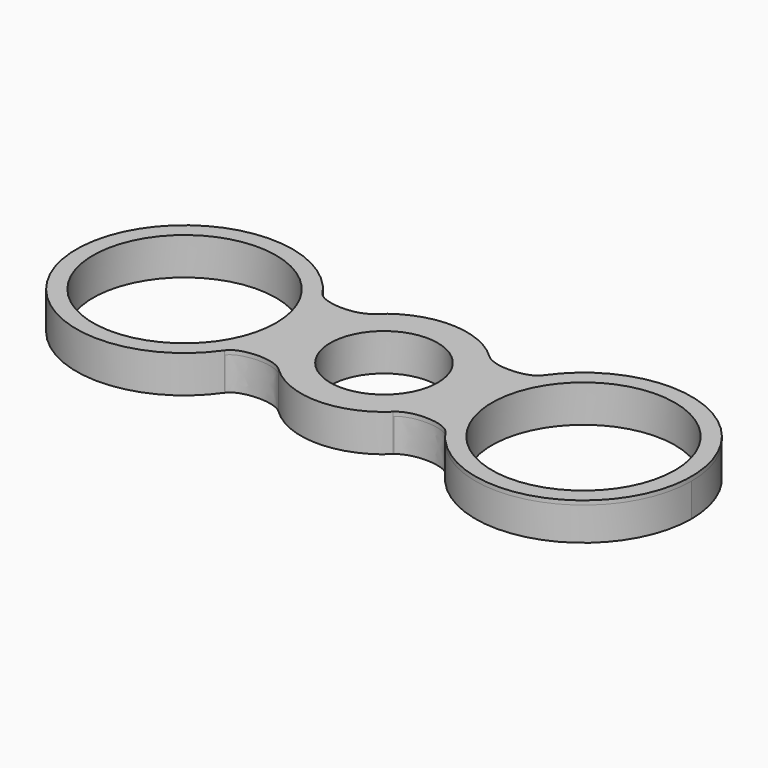
from build123d import *

# Parameters (mm, degrees)
F0_R        = 11.025
F0_R_2      = 8
F0_R_3      = 6.475
F1_DEPTH    = 4
F2_DEPTH    = 4.5
F1_FACE_R   = 11.025
F1_FACE_R_2 = 8
F3_DEPTH    = 0.5


# Not quite as in the source:
# - a feature names something its author has since deleted; it is built from what else it names


with BuildPart() as f1:
    # F0 (on Top) → F1 (new body)
    with BuildSketch(Plane.XY):
        with BuildLine():
            add(Edge.make_bspline(
                [(-13.2970699227, 7.3866190681), (-13.2858031983, 7.3692786835), (-13.2740607617, 7.352142708), (-13.2618542065, 7.3352108101)],
                knots=[0, 0, 0, 0, 0.0117546856, 0.0117546856, 0.0117546856, 0.0117546856], degree=3))
            ThreePointArc((-13.2970699227, 7.3866190681), (-37.05, 0), (-13.2970699227, -7.3866190681))
            add(Edge.make_bspline(
                [(-13.2970699227, -7.3866190681), (-13.2858031983, -7.3692786835), (-13.2740607617, -7.352142708), (-13.2618542065, -7.3352108101)],
                knots=[0, 0, 0, 0, 0.0117546856, 0.0117546856, 0.0117546856, 0.0117546856], degree=3))
            ThreePointArc((-13.2618542065, -7.3352108101), (-11.5783016635, -3.8380106201), (-11, 0))
            ThreePointArc((-11, 0), (-11.5783016635, 3.8380106201), (-13.2618542065, 7.3352108101))
        make_face()
        with Locations((-24.025, 0)):
            Circle(F0_R, mode=Mode.SUBTRACT)
        with BuildLine():
            add(Edge.make_bspline(
                [(13.2970699227, 7.3866190681), (13.2858031983, 7.3692786835), (13.2740607617, 7.352142708), (13.2618542065, 7.3352108101)],
                knots=[0, 0, 0, 0, 0.0117546856, 0.0117546856, 0.0117546856, 0.0117546856], degree=3))
            ThreePointArc((13.2618542065, 7.3352108101), (11, 0), (13.2618542065, -7.3352108101))
            add(Edge.make_bspline(
                [(13.2970699227, -7.3866190681), (13.2858031983, -7.3692786835), (13.2740607617, -7.352142708), (13.2618542065, -7.3352108101)],
                knots=[0, 0, 0, 0, 0.0117546856, 0.0117546856, 0.0117546856, 0.0117546856], degree=3))
            ThreePointArc((13.2970699227, -7.3866190681), (27.8927729861, -12.4374819448), (37.05, 0))
            ThreePointArc((37.05, 0), (27.8927729861, 12.4374819448), (13.2970699227, 7.3866190681))
        make_face()
        with Locations((24.025, 0)):
            Circle(F0_R, mode=Mode.SUBTRACT)
        with BuildLine():
            add(Edge.make_bspline(
                [(-6.9491121946, 7.1909554099), (-6.9214787847, 7.2161071506), (-6.8945995038, 7.2417846871), (-6.8685019311, 7.2679901776)],
                knots=[0.9815772058, 0.9815772058, 0.9815772058, 0.9815772058, 1, 1, 1, 1], degree=3))
            ThreePointArc((-6.9491121946, 7.1909554099), (-10, 0), (-6.9491121946, -7.1909554099))
            add(Edge.make_bspline(
                [(-6.9491121946, -7.1909554099), (-6.9214787847, -7.2161071506), (-6.8945995038, -7.2417846871), (-6.8685019311, -7.2679901776)],
                knots=[0.9815772058, 0.9815772058, 0.9815772058, 0.9815772058, 1, 1, 1, 1], degree=3))
            ThreePointArc((-6.8685019311, -7.2679901776), (0, -10), (6.8685019311, -7.2679901776))
            add(Edge.make_bspline(
                [(6.9491121946, -7.1909554099), (6.9214787847, -7.2161071506), (6.8945995038, -7.2417846871), (6.8685019311, -7.2679901776)],
                knots=[0.9815772058, 0.9815772058, 0.9815772058, 0.9815772058, 1, 1, 1, 1], degree=3))
            ThreePointArc((6.9491121946, -7.1909554099), (9.2057352217, -3.9056931558), (10, 0))
            ThreePointArc((10, 0), (9.2057352217, 3.9056931558), (6.9491121946, 7.1909554099))
            add(Edge.make_bspline(
                [(6.9491121946, 7.1909554099), (6.9214787847, 7.2161071506), (6.8945995038, 7.2417846871), (6.8685019311, 7.2679901776)],
                knots=[0.9815772058, 0.9815772058, 0.9815772058, 0.9815772058, 1, 1, 1, 1], degree=3))
            ThreePointArc((6.8685019311, 7.2679901776), (0, 10), (-6.8685019311, 7.2679901776))
        make_face()
        Circle(F0_R_2, mode=Mode.SUBTRACT)
        Circle(F0_R_2)
        Circle(F0_R_3, mode=Mode.SUBTRACT)
        with BuildLine():
            add(Edge.make_bspline(
                [(-13.2618542065, 7.3352108101), (-12.765654406, 6.6469245328), (-10.2019626219, 5.934402015), (-7.687078337, 6.5192636743), (-6.9491121946, 7.1909554099)],
                knots=[0.0117546856, 0.0117546856, 0.0117546856, 0.0117546856, 0.4895858662, 0.9815772058, 0.9815772058, 0.9815772058, 0.9815772058], degree=3))
            ThreePointArc((-13.2618542065, 7.3352108101), (-11.5783016635, 3.8380106201), (-11, 0))
            ThreePointArc((-11, 0), (-11.5783016635, -3.8380106201), (-13.2618542065, -7.3352108101))
            add(Edge.make_bspline(
                [(-13.2618542065, -7.3352108101), (-12.765654406, -6.6469245328), (-10.2019626219, -5.934402015), (-7.687078337, -6.5192636743), (-6.9491121946, -7.1909554099)],
                knots=[0.0117546856, 0.0117546856, 0.0117546856, 0.0117546856, 0.4895858662, 0.9815772058, 0.9815772058, 0.9815772058, 0.9815772058], degree=3))
            ThreePointArc((-6.9491121946, -7.1909554099), (-10, 0), (-6.9491121946, 7.1909554099))
        make_face()
        with BuildLine():
            add(Edge.make_bspline(
                [(13.2618542065, 7.3352108101), (12.765654406, 6.6469245328), (10.2019626219, 5.934402015), (7.687078337, 6.5192636743), (6.9491121946, 7.1909554099)],
                knots=[0.0117546856, 0.0117546856, 0.0117546856, 0.0117546856, 0.4895858662, 0.9815772058, 0.9815772058, 0.9815772058, 0.9815772058], degree=3))
            ThreePointArc((6.9491121946, 7.1909554099), (9.2057352217, 3.9056931558), (10, 0))
            ThreePointArc((10, 0), (9.2057352217, -3.9056931558), (6.9491121946, -7.1909554099))
            add(Edge.make_bspline(
                [(13.2618542065, -7.3352108101), (12.765654406, -6.6469245328), (10.2019626219, -5.934402015), (7.687078337, -6.5192636743), (6.9491121946, -7.1909554099)],
                knots=[0.0117546856, 0.0117546856, 0.0117546856, 0.0117546856, 0.4895858662, 0.9815772058, 0.9815772058, 0.9815772058, 0.9815772058], degree=3))
            ThreePointArc((13.2618542065, -7.3352108101), (11, 0), (13.2618542065, 7.3352108101))
        make_face()
    extrude(amount=F1_DEPTH)

    # F0 (on Top) → F2 (join)
    with BuildSketch(Plane.XY):
        Circle(F0_R_2)
        Circle(F0_R_3, mode=Mode.SUBTRACT)
    extrude(amount=F2_DEPTH)

    # F1_face (on face) + F0 (on Top) → F3 (join, through all)
    with BuildSketch(Plane.XY.offset(4)):
        with BuildLine():
            ThreePointArc((-6.8685019311, -7.2679901776), (0, -10), (6.8685019311, -7.2679901776))
            add(Edge.make_bspline(
                [(6.8685019311, -7.2679901776), (7.591550229, -6.5419519543), (10.1837329047, -5.9134794065), (12.8278077735, -6.6643873129), (13.2970699227, -7.3866190681)],
                knots=[0.9815772058, 0.9815772058, 0.9815772058, 0.9815772058, 1.4919913396, 1.9815772058, 1.9815772058, 1.9815772058, 1.9815772058], degree=3))
            ThreePointArc((13.2970699227, -7.3866190681), (37.05, 0), (13.2970699227, 7.3866190681))
            add(Edge.make_bspline(
                [(13.2970699227, 7.3866190681), (12.8278077735, 6.6643873129), (10.1837329047, 5.9134794065), (7.591550229, 6.5419519543), (6.8685019311, 7.2679901776)],
                knots=[0, 0, 0, 0, 0.4895858662, 1, 1, 1, 1], degree=3))
            ThreePointArc((6.8685019311, 7.2679901776), (0, 10), (-6.8685019311, 7.2679901776))
            add(Edge.make_bspline(
                [(-6.8685019311, 7.2679901776), (-7.591550229, 6.5419519543), (-10.1837329047, 5.9134794066), (-12.8278077735, 6.6643873129), (-13.2970699227, 7.3866190681)],
                knots=[0.9815772058, 0.9815772058, 0.9815772058, 0.9815772058, 1.4919913396, 1.9815772058, 1.9815772058, 1.9815772058, 1.9815772058], degree=3))
            ThreePointArc((-13.2970699227, 7.3866190681), (-37.05, 0), (-13.2970699227, -7.3866190681))
            add(Edge.make_bspline(
                [(-13.2970699227, -7.3866190681), (-12.8278077735, -6.6643873129), (-10.1837329047, -5.9134794065), (-7.591550229, -6.5419519543), (-6.8685019311, -7.2679901776)],
                knots=[0, 0, 0, 0, 0.4895858662, 1, 1, 1, 1], degree=3))
        make_face()
        with Locations((-24.025, 0)):
            Circle(F1_FACE_R, mode=Mode.SUBTRACT)
        Circle(F1_FACE_R_2, mode=Mode.SUBTRACT)
        with Locations((24.025, 0)):
            Circle(F1_FACE_R, mode=Mode.SUBTRACT)
    with BuildSketch(Plane.XY):
        with BuildLine():
            add(Edge.make_bspline(
                [(-13.2970699227, 7.3866190681), (-13.2858031983, 7.3692786835), (-13.2740607617, 7.352142708), (-13.2618542065, 7.3352108101)],
                knots=[0, 0, 0, 0, 0.0117546856, 0.0117546856, 0.0117546856, 0.0117546856], degree=3))
            ThreePointArc((-13.2970699227, 7.3866190681), (-37.05, 0), (-13.2970699227, -7.3866190681))
            add(Edge.make_bspline(
                [(-13.2970699227, -7.3866190681), (-13.2858031983, -7.3692786835), (-13.2740607617, -7.352142708), (-13.2618542065, -7.3352108101)],
                knots=[0, 0, 0, 0, 0.0117546856, 0.0117546856, 0.0117546856, 0.0117546856], degree=3))
            ThreePointArc((-13.2618542065, -7.3352108101), (-11.5783016635, -3.8380106201), (-11, 0))
            ThreePointArc((-11, 0), (-11.5783016635, 3.8380106201), (-13.2618542065, 7.3352108101))
        make_face()
        with Locations((-24.025, 0)):
            Circle(F0_R, mode=Mode.SUBTRACT)
        with BuildLine():
            add(Edge.make_bspline(
                [(-13.2618542065, 7.3352108101), (-12.765654406, 6.6469245328), (-10.2019626219, 5.934402015), (-7.687078337, 6.5192636743), (-6.9491121946, 7.1909554099)],
                knots=[0.0117546856, 0.0117546856, 0.0117546856, 0.0117546856, 0.4895858662, 0.9815772058, 0.9815772058, 0.9815772058, 0.9815772058], degree=3))
            ThreePointArc((-13.2618542065, 7.3352108101), (-11.5783016635, 3.8380106201), (-11, 0))
            ThreePointArc((-11, 0), (-11.5783016635, -3.8380106201), (-13.2618542065, -7.3352108101))
            add(Edge.make_bspline(
                [(-13.2618542065, -7.3352108101), (-12.765654406, -6.6469245328), (-10.2019626219, -5.934402015), (-7.687078337, -6.5192636743), (-6.9491121946, -7.1909554099)],
                knots=[0.0117546856, 0.0117546856, 0.0117546856, 0.0117546856, 0.4895858662, 0.9815772058, 0.9815772058, 0.9815772058, 0.9815772058], degree=3))
            ThreePointArc((-6.9491121946, -7.1909554099), (-10, 0), (-6.9491121946, 7.1909554099))
        make_face()
        with BuildLine():
            add(Edge.make_bspline(
                [(-6.9491121946, 7.1909554099), (-6.9214787847, 7.2161071506), (-6.8945995038, 7.2417846871), (-6.8685019311, 7.2679901776)],
                knots=[0.9815772058, 0.9815772058, 0.9815772058, 0.9815772058, 1, 1, 1, 1], degree=3))
            ThreePointArc((-6.9491121946, 7.1909554099), (-10, 0), (-6.9491121946, -7.1909554099))
            add(Edge.make_bspline(
                [(-6.9491121946, -7.1909554099), (-6.9214787847, -7.2161071506), (-6.8945995038, -7.2417846871), (-6.8685019311, -7.2679901776)],
                knots=[0.9815772058, 0.9815772058, 0.9815772058, 0.9815772058, 1, 1, 1, 1], degree=3))
            ThreePointArc((-6.8685019311, -7.2679901776), (0, -10), (6.8685019311, -7.2679901776))
            add(Edge.make_bspline(
                [(6.9491121946, -7.1909554099), (6.9214787847, -7.2161071506), (6.8945995038, -7.2417846871), (6.8685019311, -7.2679901776)],
                knots=[0.9815772058, 0.9815772058, 0.9815772058, 0.9815772058, 1, 1, 1, 1], degree=3))
            ThreePointArc((6.9491121946, -7.1909554099), (9.2057352217, -3.9056931558), (10, 0))
            ThreePointArc((10, 0), (9.2057352217, 3.9056931558), (6.9491121946, 7.1909554099))
            add(Edge.make_bspline(
                [(6.9491121946, 7.1909554099), (6.9214787847, 7.2161071506), (6.8945995038, 7.2417846871), (6.8685019311, 7.2679901776)],
                knots=[0.9815772058, 0.9815772058, 0.9815772058, 0.9815772058, 1, 1, 1, 1], degree=3))
            ThreePointArc((6.8685019311, 7.2679901776), (0, 10), (-6.8685019311, 7.2679901776))
        make_face()
        Circle(F0_R_2, mode=Mode.SUBTRACT)
    extrude(amount=F3_DEPTH)


solid = f1.part
